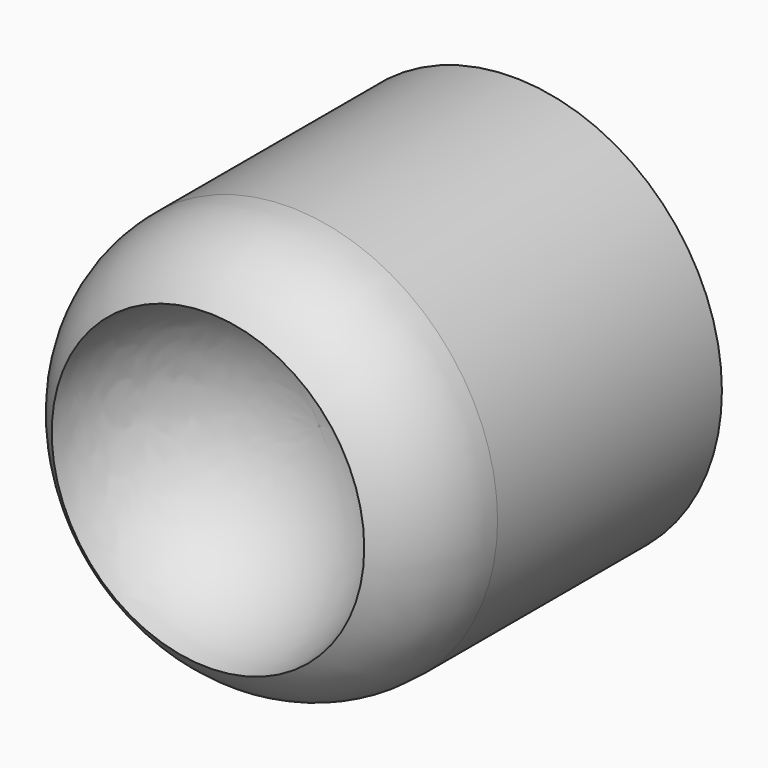
from build123d import *

# Parameters (mm, degrees)
F0_R     = 38.1
F1_DEPTH = 69.85
F2_R     = 28.575
F3_DEPTH = 25.4


# Not quite as in the source:
# - a fillet or chamfer that OpenCascade refuses, or shapes differently, is made with other operations: its cross-section is extruded or revolved along the edge and cut away or added


with BuildPart() as f1:
    # F0 (on Front) → F1 (new body)
    with BuildSketch(Plane.XZ):
        Circle(F0_R)
    extrude(amount=F1_DEPTH)

    # F2 (on face) → F3 (cut)
    with BuildSketch(Plane.XZ.offset(69.85)):
        Circle(F2_R)
    extrude(amount=-F3_DEPTH, mode=Mode.SUBTRACT)

    # F4: fillet of radius 28.59786 on 1 edges, made by hand

    # F4_s1 → F4_t2 (revolve)
    with BuildSketch(Plane.XY):
        with BuildLine():
            ThreePointArc((28.575, -69.85), (19.2141159123, -51.7254592304), (0.1564974356, -44.45))
            Line((0.1564974356, -44.45), (28.575, -44.45))
            Line((28.575, -44.45), (28.575, -69.85))
        make_face()
    revolve(axis=Axis((0, -44.45, 0), (0, -1, 0)))

    # F5: fillet of radius 22.86 on 1 edges, made by hand

    # F5_s1 → F5_t2 (revolve, cut)
    with BuildSketch(Plane.XY):
        with BuildLine():
            ThreePointArc((38.1, -51.2823567731), (35.5798340701, -61.7164714936), (28.575, -69.85))
            Line((28.575, -69.85), (38.1, -69.85))
            Line((38.1, -69.85), (38.1, -51.2823567731))
        make_face()
    revolve(axis=Axis((0, -69.85, 0), (0, -1, 0)), mode=Mode.SUBTRACT)


solid = f1.part
